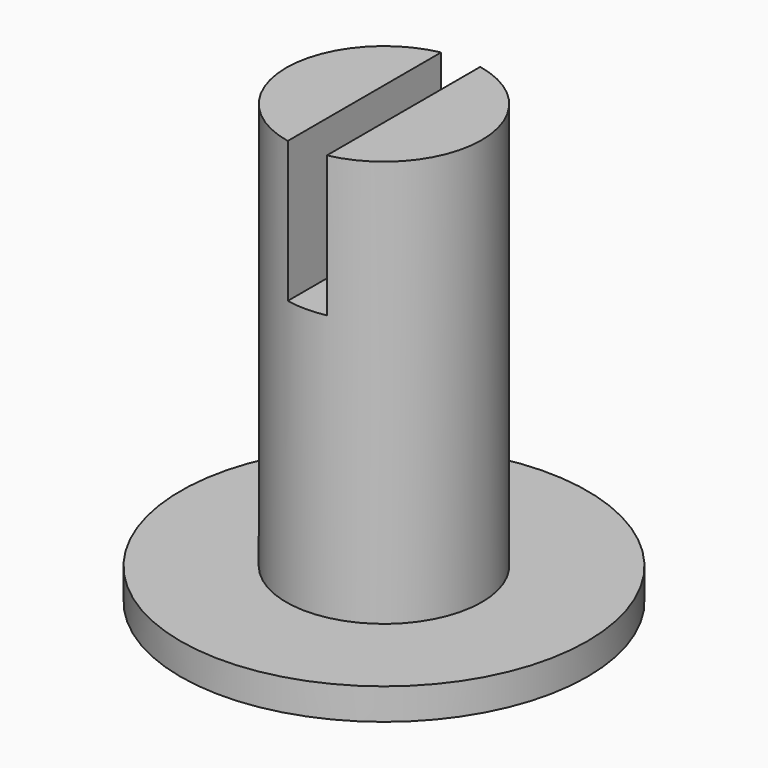
from build123d import *

# Parameters (mm, degrees)
F0_R     = 3.125
F1_DEPTH = 14
F0_R_2   = 6.5
F2_DEPTH = 1
F4_DEPTH = 4.5


with BuildPart() as f1:
    # F0 (on Top) → F1 (new body)
    with BuildSketch(Plane.XY):
        Circle(F0_R)
    extrude(amount=F1_DEPTH)

    # F0 (on Top) → F2 (join)
    with BuildSketch(Plane.XY):
        Circle(F0_R_2)
        Circle(F0_R, mode=Mode.SUBTRACT)
    extrude(amount=F2_DEPTH)

    # F3 (on face) → F4 (cut)
    with BuildSketch(Plane.XY.offset(14)):
        with BuildLine():
            Line((0.625, -3.0618621785), (0.625, 3.0618621785))
            ThreePointArc((0.625, 3.0618621785), (0, 3.125), (-0.625, 3.0618621785))
            Line((-0.625, 3.0618621785), (-0.625, -3.0618621785))
            ThreePointArc((-0.625, -3.0618621785), (0, -3.125), (0.625, -3.0618621785))
        make_face()
    extrude(amount=-F4_DEPTH, mode=Mode.SUBTRACT)


solid = f1.part
